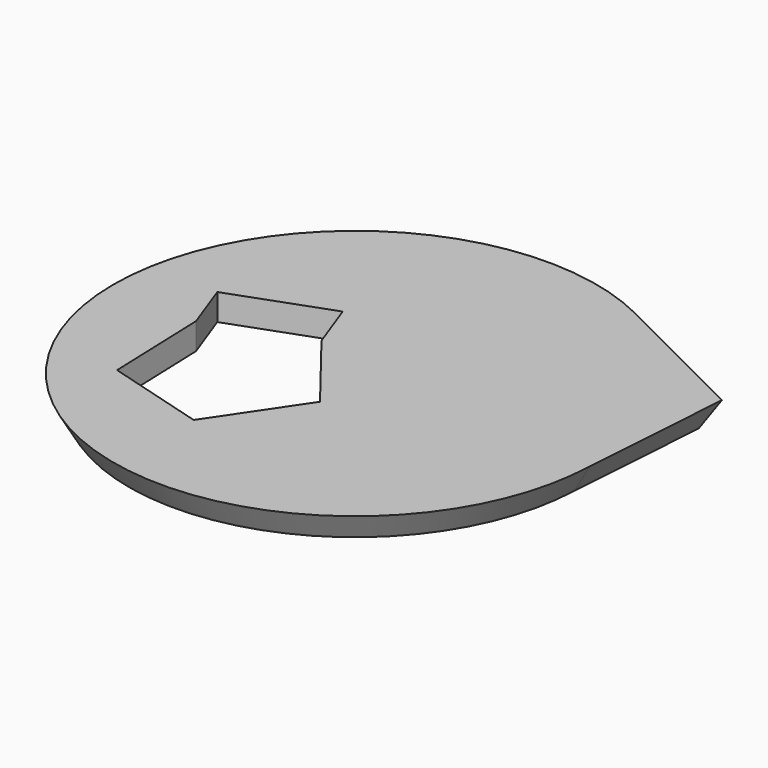
from build123d import *

# Parameters (mm, degrees)
F3_DEPTH = 25.4
F3_TAPER = -30
F5_DEPTH = 74.422
F6_DEPTH = 49.784


# Not quite as in the source:
# - the program builds the solid bodies; features that only make, move or delete a surface that nothing else refers to are left out


with BuildPart() as f3:
    # F2 (on Top) → F3 (new body)
    with BuildSketch(Plane.XY):
        with BuildLine():
            ThreePointArc((95.3163852149, 108.891700447), (-188.3047271115, -196.2747006031), (215.153157711, -92.4036128949))
            Line((215.153157711, -92.4036128949), (224.725946784, 44.1582836211))
            Line((224.725946784, 44.1582836211), (95.3163852149, 108.891700447))
        make_face()
    extrude(amount=F3_DEPTH, taper=F3_TAPER)

    # F4 (on face) → F5 (cut)
    with BuildSketch(Plane.XY.offset(25.4)):
        Polygon((-144.5069598745, -192.3162760185), (-49.1051686216, -219.640064056), (6.3620728322, -137.351083673), (-54.75907794, -59.1699088592), (-148.0012680026, -93.1402659269), align=None)
    extrude(amount=-F5_DEPTH, mode=Mode.SUBTRACT)

    # F6 (cut): a face of the model
    f6_faces = [f3.faces().sort_by_distance(p)[0] for p in [
        (-101.3801729713, -76.1550873931, 12.7),
    ]]
    extrude(f6_faces, amount=-F6_DEPTH, mode=Mode.SUBTRACT)


solid = f3.part
